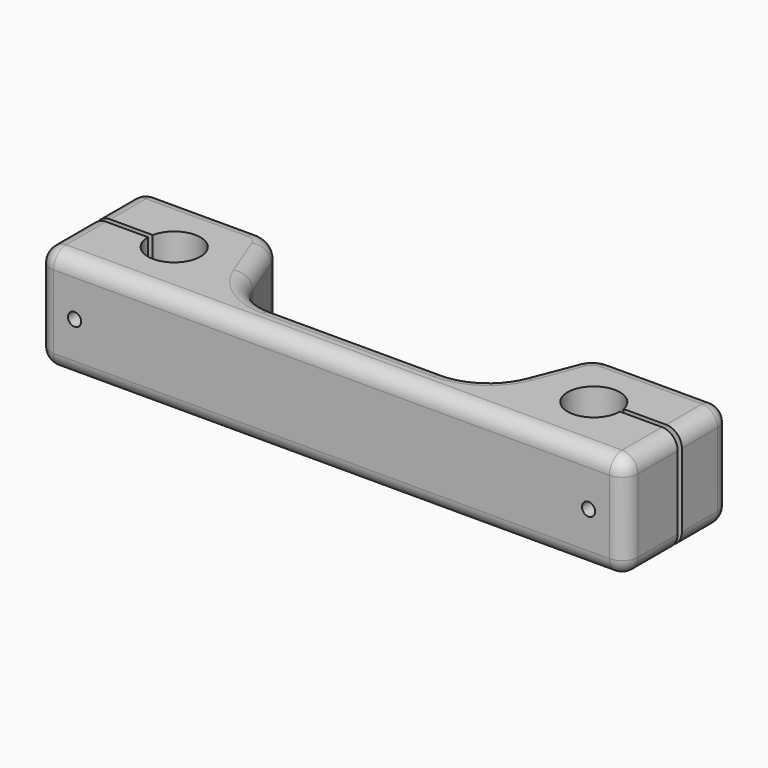
from build123d import *

# Parameters (mm, degrees)
F1_DEPTH  = 20
F2_R      = 3
F3_R      = 1.25
F4_DEPTH  = 30
F3_R_2    = 1.75
F5_DEPTH  = 12
F3_R_3    = 3.5
F6_DEPTH  = 4
F7_R      = 1.25
F8_DEPTH  = 30
F7_R_2    = 1.75
F9_DEPTH  = 12
F7_R_3    = 3.5
F10_DEPTH = 4


# Not quite as in the source:
# - a feature names something its author has since deleted; it is built from what else it names


with BuildPart() as f1:
    # F0 (on Top) → F1 (new body)
    with BuildSketch(Plane.XY):
        with BuildLine():
            Line((3, 0), (56, 0))
            Line((56, 0), (109, 0))
            ThreePointArc((109, 0), (111.1213203436, 0.8786796564), (112, 3))
            Line((112, 3), (112, 12.5))
            Line((112, 12.5), (101, 12.5))
            ThreePointArc((101, 12.5), (91.025319235, 11.99745519), (100.8989794856, 13.5))
            Line((100.8989794856, 13.5), (112, 13.5))
            Line((112, 13.5), (112, 22))
            ThreePointArc((112, 22), (111.1213203436, 24.1213203436), (109, 25))
            Line((109, 25), (95.7940161003, 25))
            Line((95.7940161003, 25), (92, 25))
            Line((92, 25), (89.649228215, 25))
            ThreePointArc((89.649228215, 25), (86.8322254301, 24.1309194267), (84.9945036033, 21.825798124))
            Line((84.9945036033, 21.825798124), (81.660193975, 13.3252454689))
            ThreePointArc((81.660193975, 13.3252454689), (77.9847503214, 8.7150028635), (72.3507447516, 6.9768417168))
            Line((72.3507447516, 6.9768417168), (61.9619729666, 6.9768417168))
            Line((61.9619729666, 6.9768417168), (56, 6.9768417168))
            Line((56, 6.9768417168), (50.0380270334, 6.9768417168))
            Line((50.0380270334, 6.9768417168), (39.6492552484, 6.9768417168))
            ThreePointArc((39.6492552484, 6.9768417168), (34.0152496786, 8.7150028635), (30.339806025, 13.3252454689))
            Line((30.339806025, 13.3252454689), (27.0054963967, 21.825798124))
            ThreePointArc((27.0054963967, 21.825798124), (25.1677745699, 24.1309194267), (22.350771785, 25))
            Line((22.350771785, 25), (20, 25))
            Line((20, 25), (16.2059838997, 25))
            Line((16.2059838997, 25), (3, 25))
            ThreePointArc((3, 25), (0.8786796564, 24.1213203436), (0, 22))
            Line((0, 22), (0, 13.5))
            Line((0, 13.5), (11.1010205144, 13.5))
            ThreePointArc((11.1010205144, 13.5), (20.974680765, 11.99745519), (11, 12.5))
            Line((11, 12.5), (0, 12.5))
            Line((0, 12.5), (0, 3))
            ThreePointArc((0, 3), (0.8786796564, 0.8786796564), (3, 0))
        make_face()
    extrude(amount=F1_DEPTH)

    # F2
    f2_edges = [f1.edges().sort_by_distance(p)[0] for p in [
        (56, 0, 20),
        (99.324614, 25, 20),
        (56, 0, 0),
        (99.324614, 25, 0),
    ]]
    fillet(f2_edges, radius=F2_R)

    # F3 (on face) → F4 (cut)
    with BuildSketch(Plane(origin=(0, 25, 0), x_dir=(-1, 0, 0), z_dir=(0, 1, 0))):
        with Locations((-7, 10)):
            Circle(F3_R)
    extrude(amount=-F4_DEPTH, mode=Mode.SUBTRACT)

    # F3 (on face) → F5 (cut)
    with BuildSketch(Plane(origin=(0, 25, 0), x_dir=(-1, 0, 0), z_dir=(0, 1, 0))):
        with Locations((-7, 10)):
            Circle(F3_R_2)
        with Locations((-7, 10)):
            Circle(F3_R, mode=Mode.SUBTRACT)
    extrude(amount=-F5_DEPTH, mode=Mode.SUBTRACT)

    # F3 (on face) → F6 (cut)
    with BuildSketch(Plane(origin=(0, 25, 0), x_dir=(-1, 0, 0), z_dir=(0, 1, 0))):
        with Locations((-7, 10)):
            Circle(F3_R_3)
        with Locations((-7, 10)):
            Circle(F3_R_2, mode=Mode.SUBTRACT)
        with Locations((-7, 10)):
            Circle(F3_R_2)
        with Locations((-7, 10)):
            Circle(F3_R, mode=Mode.SUBTRACT)
        with Locations((-7, 10)):
            Circle(F3_R)
    extrude(amount=-F6_DEPTH, mode=Mode.SUBTRACT)

    # F7 (on face) → F8 (cut)
    with BuildSketch(Plane(origin=(0, 25, 0), x_dir=(-1, 0, 0), z_dir=(0, 1, 0))):
        with Locations((-105, 10)):
            Circle(F7_R)
    extrude(amount=-F8_DEPTH, mode=Mode.SUBTRACT)

    # F7 (on face) → F9 (cut)
    with BuildSketch(Plane(origin=(0, 25, 0), x_dir=(-1, 0, 0), z_dir=(0, 1, 0))):
        with Locations((-105, 10)):
            Circle(F7_R_2)
        with Locations((-105, 10)):
            Circle(F7_R, mode=Mode.SUBTRACT)
    extrude(amount=-F9_DEPTH, mode=Mode.SUBTRACT)

    # F7 (on face) → F10 (cut)
    with BuildSketch(Plane(origin=(0, 25, 0), x_dir=(-1, 0, 0), z_dir=(0, 1, 0))):
        with Locations((-105, 10)):
            Circle(F7_R_3)
        with Locations((-105, 10)):
            Circle(F7_R_2, mode=Mode.SUBTRACT)
    extrude(amount=-F10_DEPTH, mode=Mode.SUBTRACT)


solid = f1.part
